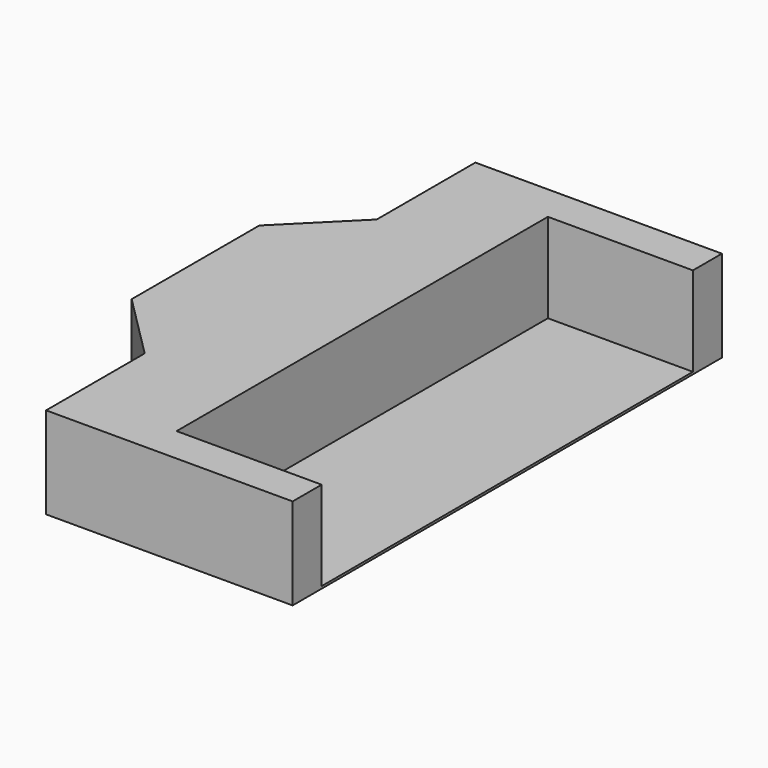
from build123d import *

# Parameters (mm, degrees)
F0_W     = 1.905
F0_H     = 8.89
F1_DEPTH = 7.62
F3_DEPTH = 0.4
F4_W     = 12.7
F4_H     = 40.64
F5_DEPTH = 0.2
F6_SIZE  = 5.71499


# Not quite as in the source:
# - a fillet or chamfer is up to 0.001 mm smaller than in the source, because OpenCascade refuses the exact size


with BuildPart() as f1:
    # F0 (on Top) → F1 (new body)
    with BuildSketch(Plane.XY):
        Polygon((-14.605, 6.985), (-14.605, 0), (-14.605, -6.985), (-8.89, -6.985), (-8.89, -23.495), (12.7, -23.495), (12.7, -20.32), (0, -20.32), (0, 0), (0, 20.32), (12.7, 20.32), (12.7, 23.495), (-8.89, 23.495), (-8.89, 6.985), align=None)
        with Locations((-11.1125, 0)):
            Rectangle(F0_W, F0_H, mode=Mode.SUBTRACT)
    extrude(amount=F1_DEPTH)

    # F2 (on face) → F3 (join)
    with BuildSketch(Plane.XY.offset(7.62)):
        Polygon((0, -20.32), (0, 20.32), (12.7, 20.32), (12.7, 23.495), (-8.89, 23.495), (-8.89, 6.985), (-14.605, 6.985), (-14.605, -6.985), (-8.89, -6.985), (-8.89, -23.495), (12.7, -23.495), (12.7, -20.32), align=None)
    extrude(amount=F3_DEPTH)

    # F4 (on face) → F5 (join)
    with BuildSketch(Plane(origin=(0, 0, 0), x_dir=(1, 0, 0), z_dir=(0, 0, -1))):
        with Locations((6.35, 0)):
            Rectangle(F4_W, F4_H)
    extrude(amount=-F5_DEPTH)

    # F6 (size 5.715 in the source; OpenCascade refuses exactly that, so slightly less here)
    f6_edges = [f1.edges().sort_by_distance(p)[0] for p in [
        (-8.89, 6.985, 4.01),
        (-8.89, -6.985, 4.01),
    ]]
    chamfer(f6_edges, length=F6_SIZE)


solid = f1.part
